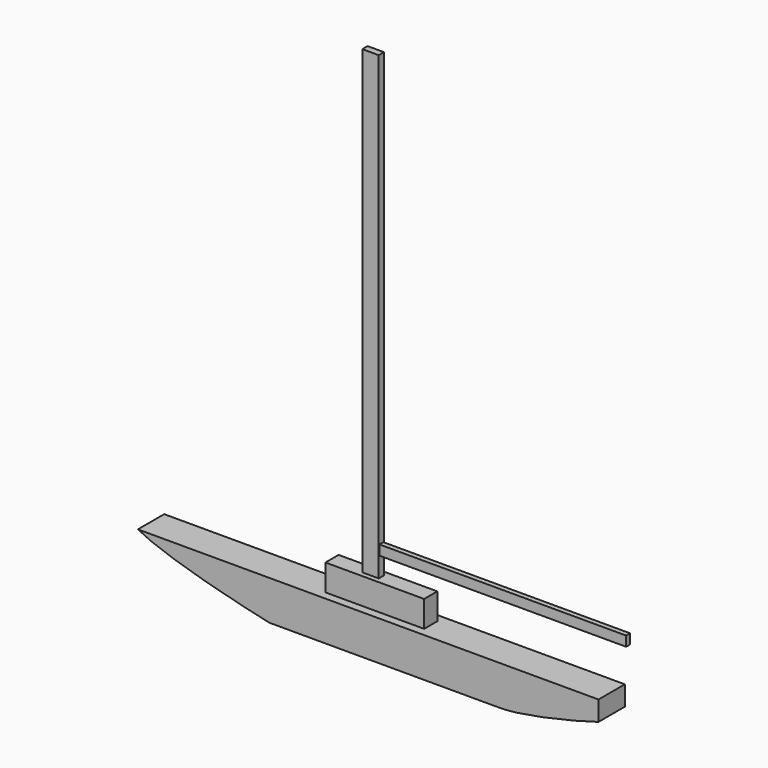
from build123d import *

# Parameters (mm, degrees)
F1_DEPTH = 12.7
F2_DEPTH = 2.54
F0_W     = 190.5
F0_H     = 7.62
F3_DEPTH = 1.905
F4_DEPTH = 6.35
F5_W     = 50.8
F5_H     = 17.78
F6_DEPTH = 10.16


# Not quite as in the source:
# - a feature names something its author has since deleted; it is built from what else it names


with BuildPart() as f1:
    # F0 (on Front) → F1 (new body, symmetric)
    with BuildSketch(Plane.XZ):
        Polygon((114.3, -15.24), (114.3, 15.24), (50.8, 15.24), (-25.4, 15.24), (-63.5, 15.24), (-63.5, -15.24), align=None)
        with BuildLine():
            add(Edge.make_bspline(
                [(-165.1, 15.24), (-140.9795414875, 2.2073420069), (-78.9946019822, -11.9854301172), (-63.5, -15.24)],
                knots=[0, 0, 0, 0, 106.0735141305, 106.0735141305, 106.0735141305, 106.0735141305], degree=3))
            Line((-63.5, -15.24), (-63.5, 15.24))
            Line((-63.5, 15.24), (-165.1, 15.24))
        make_face()
        with BuildLine():
            Line((190.5, 15.24), (114.3, 15.24))
            Line((114.3, 15.24), (114.3, -15.24))
            add(Edge.make_bspline(
                [(190.5, 0), (180.2725183696, -3.34228636), (135.7526859203, -15.2111054963), (114.3, -15.24)],
                knots=[0, 0, 0, 0, 77.7090573872, 77.7090573872, 77.7090573872, 77.7090573872], degree=3))
            Line((190.5, 0), (190.5, 15.24))
        make_face()
    extrude(amount=F1_DEPTH, both=True)

    # F5 (on Top) → F6 (cut)
    with BuildSketch(Plane.XY):
        with Locations((154.94, 0)):
            Rectangle(F5_W, F5_H)
    extrude(amount=F6_DEPTH, mode=Mode.SUBTRACT)


with BuildPart() as f2:
    # F0 (on Front) → F2 (new body, symmetric)
    with BuildSketch(Plane.XZ):
        Polygon((0, 35.56), (12.7, 35.56), (12.7, 50.8), (12.7, 58.42), (12.7, 391.16), (0, 391.16), align=None)
    extrude(amount=F2_DEPTH, both=True)


with BuildPart() as f3:
    # F0 (on Front) → F3 (new body, symmetric)
    with BuildSketch(Plane.XZ):
        with Locations((107.95, 54.61)):
            Rectangle(F0_W, F0_H)
    extrude(amount=F3_DEPTH, both=True)


with BuildPart() as f4:
    # F0 (on Front) → F4 (new body, symmetric)
    with BuildSketch(Plane.XZ):
        Polygon((-25.4, 15.24), (50.8, 15.24), (50.8, 35.56), (12.7, 35.56), (0, 35.56), (-25.4, 35.56), align=None)
    extrude(amount=F4_DEPTH, both=True)


solid = Compound([f1.part, f2.part, f3.part, f4.part])
